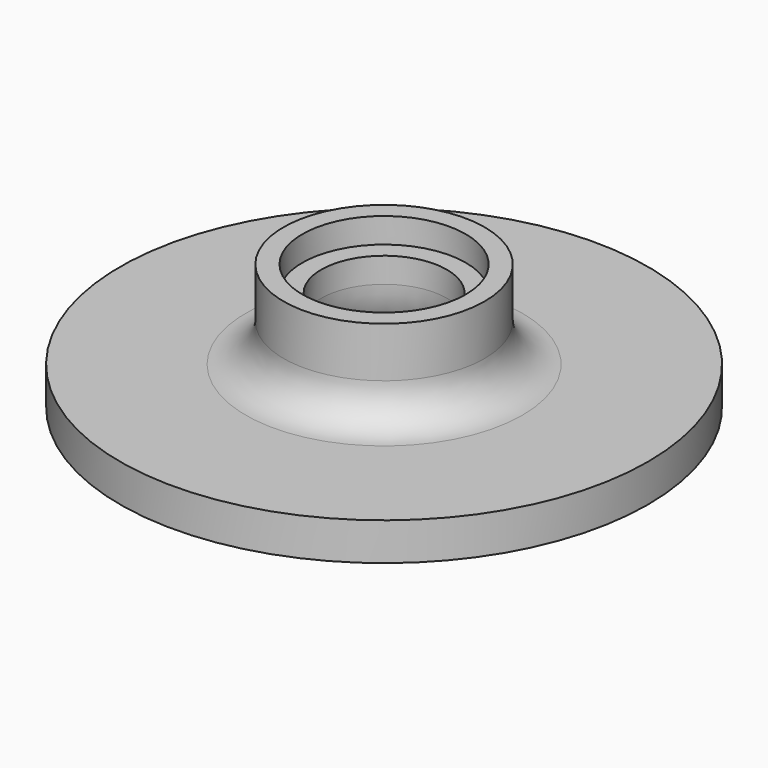
from build123d import *

# Parameters (mm, degrees)
F0_W = 1.5
F0_H = 2


# Not quite as in the source:
# - a feature names something its author has since deleted; it is built from what else it names


with BuildPart() as f2:
    # F0 (on Front) → F2 (revolve)
    with BuildSketch(Plane.XZ):
        with BuildLine():
            Line((6.5, 8), (5, 8))
            Line((5, 8), (5, 6))
            ThreePointArc((5, 6), (6.7573593129, 1.7573593129), (11, 0))
            Line((11, 0), (21, 0))
            Line((21, 0), (21, 3))
            Line((21, 3), (11, 3))
            ThreePointArc((11, 3), (8.8786796564, 3.8786796564), (8, 6))
            Line((8, 6), (8, 8))
            Line((8, 8), (6.5, 8))
        make_face()
        with Locations((7.25, 9)):
            Rectangle(F0_W, F0_H)
    revolve(axis=Axis((0, 0, 0), (0, 0, 1)))


solid = f2.part
